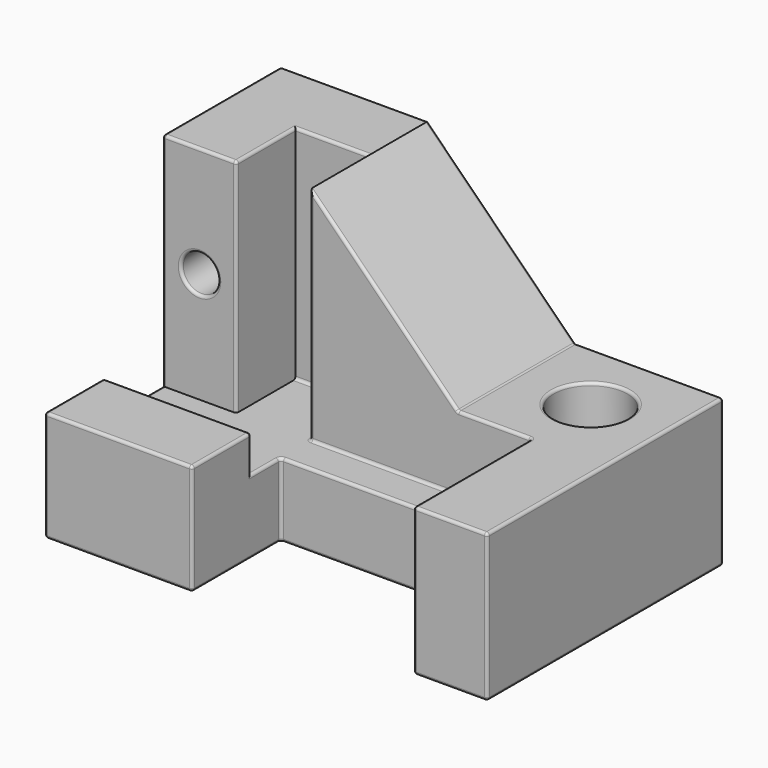
from build123d import *

# Parameters (mm, degrees)
F0_W      = 50
F0_H      = 150
F1_DEPTH  = 50
F2_DEPTH  = 100
F3_DEPTH  = 125
F4_DEPTH  = 200
F6_DEPTH  = 100
F7_R      = 12.5
F8_DEPTH  = 100.001
F9_R      = 25
F10_DEPTH = 100.001
F11_R     = 1.9


# Not quite as in the source:
# - a feature names something its author has since deleted; it is built from what else it names


with BuildPart() as f1:
    # F0 (on Front) → F1 (new body)
    with BuildSketch(Plane.XZ):
        with Locations((75, 125)):
            Rectangle(F0_W, F0_H)
    extrude(amount=F1_DEPTH)

    # F0 (on Front) → F2 (join)
    with BuildSketch(Plane.XZ):
        with Locations((25, 125)):
            Rectangle(F0_W, F0_H)
        Polygon((200, 50), (250, 50), (250, 100), (200, 100), (100, 200), (100, 50), align=None)
    extrude(amount=F2_DEPTH)

    # F0 (on Front) → F3 (join)
    with BuildSketch(Plane.XZ):
        Polygon((0, 50), (0, 0), (250, 0), (250, 50), (200, 50), (100, 50), (50, 50), align=None)
    extrude(amount=F3_DEPTH)

    # F0 (on Front) → F4 (join)
    with BuildSketch(Plane.XZ):
        Polygon((250, 50), (250, 0), (300, 0), (300, 50), (300, 100), (250, 100), align=None)
    extrude(amount=F4_DEPTH)

    # F5 (on Right) → F6 (join)
    with BuildSketch(Plane.YZ):
        Polygon((-125, 0), (-125, 50), (-150, 50), (-150, 75), (-200, 75), (-200, 0), align=None)
    extrude(amount=F6_DEPTH)

    # F7 (on face) → F8 (cut, through all)
    with BuildSketch(Plane.XZ.offset(100)):
        with Locations((25, 125)):
            Circle(F7_R)
    extrude(amount=-F8_DEPTH, mode=Mode.SUBTRACT)

    # F9 (on face) → F10 (cut, through all)
    with BuildSketch(Plane.XY.offset(100)):
        with Locations((250, -50)):
            Circle(F9_R)
    extrude(amount=-F10_DEPTH, mode=Mode.SUBTRACT)

    # F11
    f11_edges = [f1.edges().sort_by_distance(p)[0] for p in [
        (0, 0, 100),
        (0, -100, 0),
        (0, -125, 50),
        (0, -200, 37.5),
        (0, -175, 75),
        (0, -150, 62.5),
        (0, -100, 125),
        (0, -50, 200),
        (50, 0, 200),
        (75, -50, 200),
        (50, -75, 200),
        (25, -100, 200),
        (150, -100, 150),
        (100, -100, 125),
        (75, -50, 50),
        (50, -100, 125),
        (225, -100, 100),
        (175, -100, 50),
        (200, -50, 100),
        (250, -100, 75),
        (250, -112.5, 50),
        (250, -125, 25),
        (175, -125, 50),
        (175, -125, 0),
        (100, -125, 25),
        (100, -137.5, 50),
        (100, -150, 62.5),
        (50, -150, 75),
        (100, -175, 75),
        (50, -200, 75),
        (100, -200, 37.5),
        (100, -162.5, 0),
        (50, -200, 0),
        (300, -100, 100),
        (275, -200, 100),
        (250, -200, 50),
        (300, -200, 50),
        (275, -200, 0),
        (250, -162.5, 0),
        (300, -100, 0),
        (250, 0, 100),
        (150, 0, 150),
        (300, 0, 50),
        (150, 0, 0),
        (225, -50, 100),
        (12.5, -100, 125),
        (225, -50, 0),
        (12.5, 0, 125),
        (250, -150, 100),
        (100, -75, 50),
    ]]
    fillet(f11_edges, radius=F11_R)


solid = f1.part
